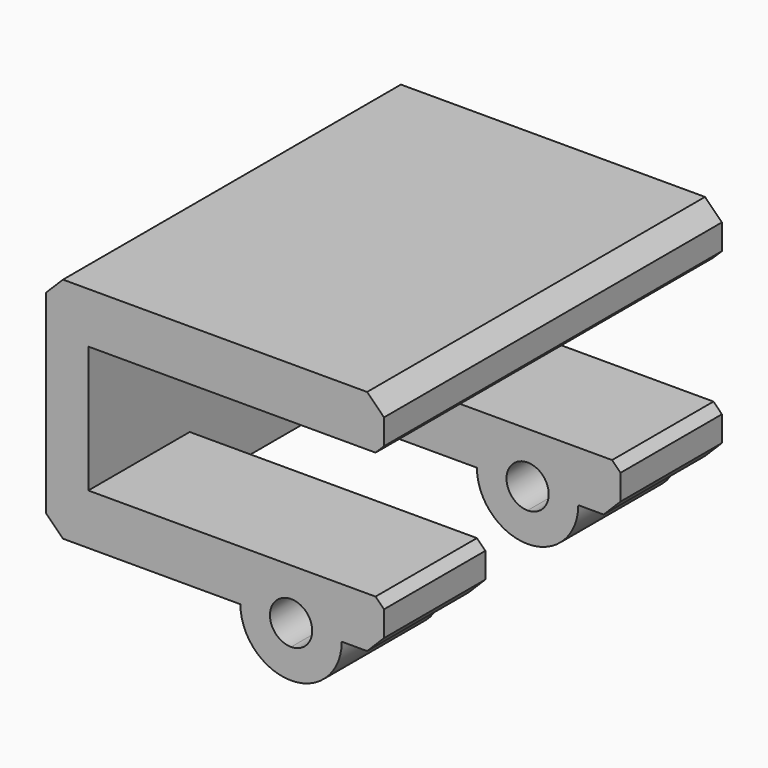
from build123d import *

# Parameters (mm, degrees)
F0_W     = 12
F0_H     = 6
F1_DEPTH = 50
F2_R     = 5.99999
F4_DEPTH = 25
F6_DEPTH = 60
F7_SIZE  = 2
F8_SIZE  = 1


# Not quite as in the source:
# - a fillet or chamfer is up to 0.001 mm smaller than in the source, because OpenCascade refuses the exact size


with BuildPart() as f1:
    # F0 (on Front) → F1 (new body)
    with BuildSketch(Plane.XZ):
        Polygon((0, 27), (0, 0), (20, 0), (23, 0), (35, 0), (40, 0), (40, 6), (5, 6), (5, 21), (40, 21), (40, 27), align=None)
        with Locations((29, -3)):
            Rectangle(F0_W, F0_H)
    extrude(amount=F1_DEPTH)

    # F2 (radius 6 in the source; OpenCascade refuses exactly that, so slightly less here)
    f2_edges = [f1.edges().sort_by_distance(p)[0] for p in [
        (23, -25, -6),
        (35, -25, -6),
    ]]
    fillet(f2_edges, radius=F2_R)

    # F3 (on face) → F4 (cut)
    with BuildSketch(Plane.XY.offset(6)):
        Polygon((40, -35), (40, -25), (40, -15), (5, -15), (5, -35), align=None)
    extrude(amount=-F4_DEPTH, mode=Mode.SUBTRACT)

    # F5 (on face) → F6 (cut)
    with BuildSketch(Plane.XZ.offset(50)):
        with BuildLine():
            ThreePointArc((29, -2.5), (30.767766953, -1.767766953), (31.5, 0))
            ThreePointArc((31.5, 0), (27.232233047, 1.767766953), (29, -2.5))
        make_face()
    extrude(amount=-F6_DEPTH, mode=Mode.SUBTRACT)

    # F7
    f7_edges = [f1.edges().sort_by_distance(p)[0] for p in [
        (0, -25, 27),
        (40, -25, 27),
        (0, -25, 0),
        (40, -42.5, 0),
        (40, -7.5, 0),
    ]]
    chamfer(f7_edges, length=F7_SIZE)

    # F8
    f8_edges = [f1.edges().sort_by_distance(p)[0] for p in [
        (40, -42.5, 6),
        (40, -7.5, 6),
        (40, -25, 21),
    ]]
    chamfer(f8_edges, length=F8_SIZE)


solid = f1.part
